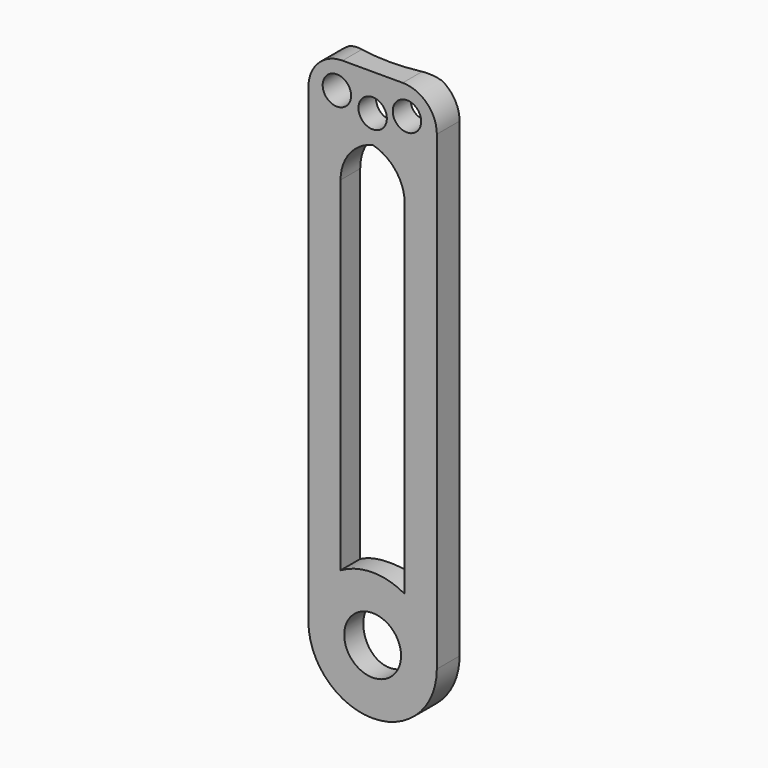
from build123d import *

# Parameters (mm, degrees)
F1_DEPTH    = 1.27
F3_D        = 2.54
F3_DEPTH    = 6.35
F3_TIP      = 0.7630929862
F4_R        = 1.524
F6_D        = 1.27
F6_DEPTH    = 6.35
F6_TIP      = 0.3815464931
F7_T1_DEPTH = 1.27
F9_D        = 13.843
F9_DEPTH    = 304.8
F9_TIP      = 4.1588567746


# Not quite as in the source:
# - a fillet or chamfer that OpenCascade refuses, or shapes differently, is made with other operations: its cross-section is extruded or revolved along the edge and cut away or added


with BuildPart() as f1:
    # F0 (on Front) → F1 (new body)
    with BuildSketch(Plane.XZ):
        with BuildLine():
            ThreePointArc((1.4341250062, 5.3522273875), (2.4839773751, 4.3023750186), (2.8682500124, 2.8682500124))
            Line((2.8682500124, 2.8682500124), (2.8682500124, 25.4276227206))
            Line((2.8682500124, 25.4276227206), (0, 25.4276227206))
            Line((0, 25.4276227206), (-1.4341250062, 25.4276227206))
            Line((-1.4341250062, 25.4276227206), (-2.8682500124, 25.4276227206))
            Line((-2.8682500124, 25.4276227206), (-2.8682500124, 2.8682500124))
            ThreePointArc((-2.8682500124, 2.8682500124), (-2.4839773751, 4.3023750186), (-1.4341250062, 5.3522273875))
            Line((-1.4341250062, 5.3522273875), (-1.4341250062, 22.6080268621))
            Line((-1.4341250062, 22.6080268621), (1.4341250062, 22.6080268621))
            Line((1.4341250062, 22.6080268621), (1.4341250062, 5.3522273875))
        make_face()
        with BuildLine():
            ThreePointArc((-2.8682500124, 2.8682500124), (0, 0), (2.8682500124, 2.8682500124))
            ThreePointArc((2.8682500124, 2.8682500124), (2.4839773751, 4.3023750186), (1.4341250062, 5.3522273875))
            ThreePointArc((1.4341250062, 5.3522273875), (0, 5.7365000248), (-1.4341250062, 5.3522273875))
            ThreePointArc((-1.4341250062, 5.3522273875), (-2.4839773751, 4.3023750186), (-2.8682500124, 2.8682500124))
        make_face()
    extrude(amount=F1_DEPTH)

    # F3
    with Locations(Plane(origin=(0, 0, 0), x_dir=(-1, 0, 0), z_dir=(0, 1, 0))):
        with Locations((0, 2.8682500124)):
            Hole(F3_D / 2, depth=F3_DEPTH)
            with Locations((0, 0, -(F3_DEPTH + F3_TIP / 2))):  # 118° drill point
                Cone(0, F3_D / 2, F3_TIP, mode=Mode.SUBTRACT)

    # F4
    f4_edges = [f1.edges().sort_by_distance(p)[0] for p in [
        (2.86825, -0.635, 25.427623),
        (-2.86825, -0.635, 25.427623),
    ]]
    fillet(f4_edges, radius=F4_R)

    # F6
    with Locations(Plane.XZ.offset(1.27)):
        with Locations((-1.5970880988, 24.1730304042), (0, 23.7946401586), (1.5335635452, 24.1730304042)):
            Hole(F6_D / 2, depth=F6_DEPTH)
            with Locations((0, 0, -(F6_DEPTH + F6_TIP / 2))):  # 118° drill point
                Cone(0, F6_D / 2, F6_TIP, mode=Mode.SUBTRACT)

    # F7: fillet of radius 1.905 on 2 edges, made by hand

    # F7_s2 → F7_t1 (join)
    with BuildSketch(Plane.XZ):
        with BuildLine():
            ThreePointArc((-0.4708749938, 22.6080268621), (0.8761634244, 22.0500652803), (1.4341250062, 20.7030268621))
            Line((1.4341250062, 20.7030268621), (1.4341250062, 22.6080268621))
            Line((1.4341250062, 22.6080268621), (-0.4708749938, 22.6080268621))
        make_face()
        with BuildLine():
            ThreePointArc((-1.4341250062, 20.7030268621), (-0.8761634244, 22.0500652803), (0.4708749938, 22.6080268621))
            Line((0.4708749938, 22.6080268621), (-1.4341250062, 22.6080268621))
            Line((-1.4341250062, 22.6080268621), (-1.4341250062, 20.7030268621))
        make_face()
    extrude(amount=F7_T1_DEPTH)

    # F9
    with Locations(Plane.XY.offset(25.4276227206)):
        with Locations((0, 6.6013582982)):
            Hole(F9_D / 2, depth=F9_DEPTH)
            with Locations((0, 0, -(F9_DEPTH + F9_TIP / 2))):  # 118° drill point
                Cone(0, F9_D / 2, F9_TIP, mode=Mode.SUBTRACT)


solid = f1.part
